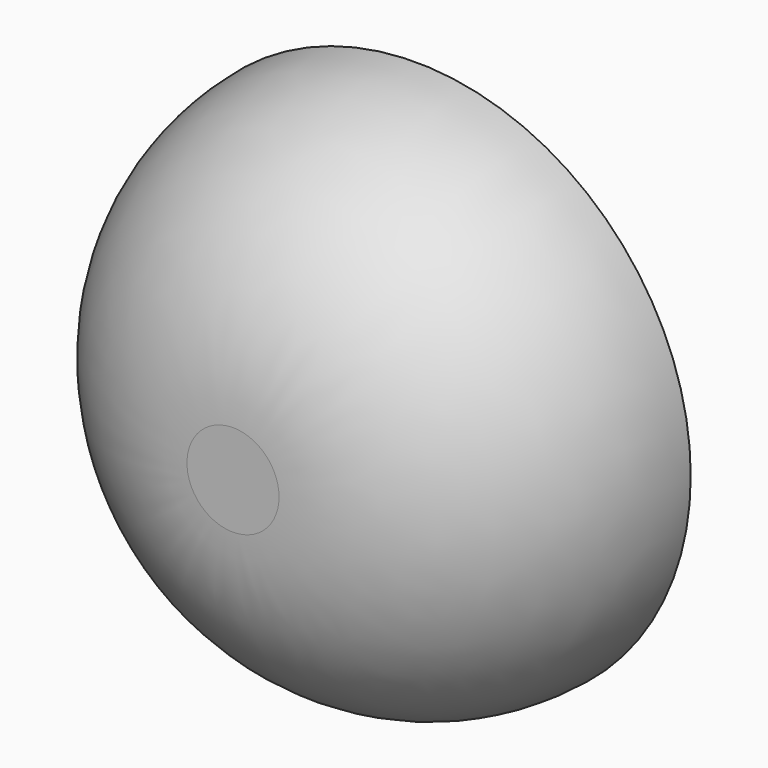
from build123d import *

# Parameters (mm, degrees)
F0_R     = 48.0560844675
F1_DEPTH = 20
F2_R     = 39.99999


# Not quite as in the source:
# - a fillet or chamfer is up to 0.001 mm smaller than in the source, because OpenCascade refuses the exact size


with BuildPart() as f1:
    # F0 (on Front) → F1 (new body, symmetric)
    with BuildSketch(Plane.XZ):
        Circle(F0_R)
    extrude(amount=F1_DEPTH, both=True)

    # F2 (radius 40 in the source; OpenCascade refuses exactly that, so slightly less here)
    f2_edges = [f1.edges().sort_by_distance(p)[0] for p in [
        (-48.056084, -20, 0),
    ]]
    fillet(f2_edges, radius=F2_R)


solid = f1.part
